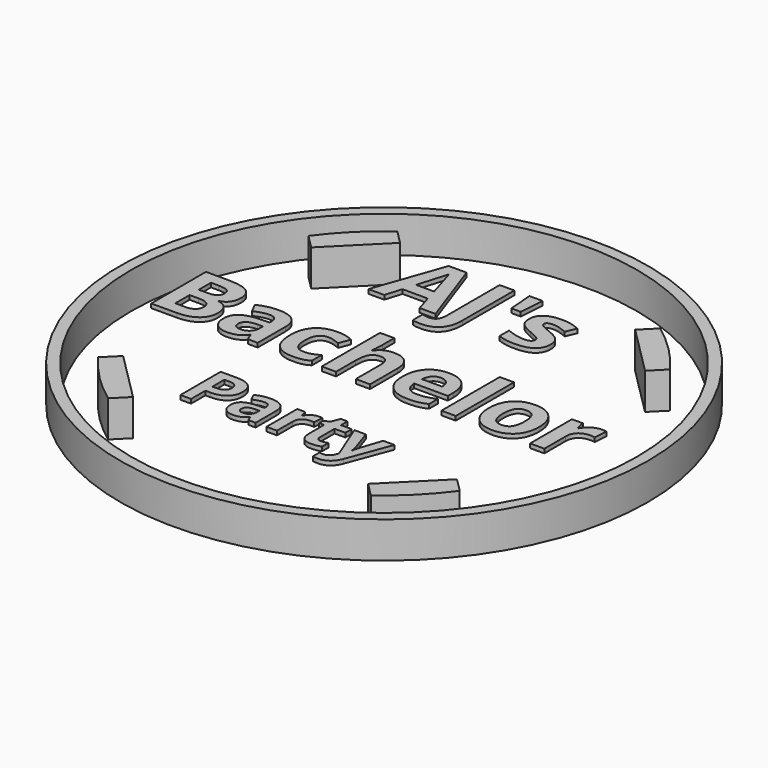
from build123d import *

# Parameters (mm, degrees)
F0_TEXT_SIZE = 8.7192851648
F1_TEXT_SIZE = 8.8355448193
F2_TEXT_SIZE = 6.411131907
F4_DEPTH     = 0.381
F5_DEPTH     = 3.302
F6_R         = 24
F6_R_2       = 23
F7_DEPTH     = 3.302


# Not quite as in the source:
# - Text() gives the source's letters only with a copy of the font that has no kerning and outlines rounded to 1/6400 em; it was checked with that copy


with BuildPart() as f4:
    # F0 (on Top) + F1 (on Top) + F2 (on Top) → F4 (new body)
    with BuildSketch(Plane.XY):
        with Locations((-19.4460495, -3.1389426593)):
            Text('Bachelor', F0_TEXT_SIZE, font='Open Sans', font_style=FontStyle.BOLD, text_align=(TextAlign.LEFT, TextAlign.BOTTOM))
    with BuildSketch(Plane.XY):
        with Locations((-8.001, 8.2189426593)):
            Text("AJ's", F1_TEXT_SIZE, font='Open Sans', font_style=FontStyle.BOLD, text_align=(TextAlign.LEFT, TextAlign.BOTTOM))
    with BuildSketch(Plane.XY):
        with Locations((-8.8278281141, -12.8349576324)):
            Text('Party', F2_TEXT_SIZE, font='Open Sans', font_style=FontStyle.BOLD, text_align=(TextAlign.LEFT, TextAlign.BOTTOM))
    extrude(amount=-F4_DEPTH)


with BuildPart() as f5:
    # F3 (on Top) → F5 (new body)
    with BuildSketch(Plane.XY):
        with BuildLine():
            Line((-16.4369943958, 11.9468663353), (-15.1766328446, 10.6865047841))
            Line((-15.1766328446, 10.6865047841), (-10.6865047841, 15.1766328446))
            Line((-10.6865047841, 15.1766328446), (-11.9468663353, 16.4369943958))
            ThreePointArc((-11.9468663353, 16.4369943958), (-14.3684097937, 14.3684097937), (-16.4369943958, 11.9468663353))
        make_face()
    extrude(amount=-F5_DEPTH)


with BuildPart() as f5b:
    # F3 (on Top) → F5, piece 2 (new body)
    with BuildSketch(Plane.XY):
        with BuildLine():
            Line((-10.6865047841, -15.1766328446), (-15.1766328446, -10.6865047841))
            Line((-15.1766328446, -10.6865047841), (-16.4369943958, -11.9468663353))
            ThreePointArc((-16.4369943958, -11.9468663353), (-14.3684097937, -14.3684097937), (-11.9468663353, -16.4369943958))
            Line((-11.9468663353, -16.4369943958), (-10.6865047841, -15.1766328446))
        make_face()
    extrude(amount=-F5_DEPTH)


with BuildPart() as f5c:
    # F3 (on Top) → F5, piece 3 (new body)
    with BuildSketch(Plane.XY):
        with BuildLine():
            Line((15.1766328446, -10.6865047841), (10.6865047841, -15.1766328446))
            Line((10.6865047841, -15.1766328446), (11.9468663353, -16.4369943958))
            ThreePointArc((11.9468663353, -16.4369943958), (14.3684097937, -14.3684097937), (16.4369943958, -11.9468663353))
            Line((16.4369943958, -11.9468663353), (15.1766328446, -10.6865047841))
        make_face()
    extrude(amount=-F5_DEPTH)


with BuildPart() as f5d:
    # F3 (on Top) → F5, piece 4 (new body)
    with BuildSketch(Plane.XY):
        with BuildLine():
            Line((10.6865047841, 15.1766328446), (15.1766328446, 10.6865047841))
            Line((15.1766328446, 10.6865047841), (16.4369943958, 11.9468663353))
            ThreePointArc((16.4369943958, 11.9468663353), (14.3684097937, 14.3684097937), (11.9468663353, 16.4369943958))
            Line((11.9468663353, 16.4369943958), (10.6865047841, 15.1766328446))
        make_face()
    extrude(amount=-F5_DEPTH)


with BuildPart() as f7:
    # F6 (on Top) → F7 (new body)
    with BuildSketch(Plane.XY):
        Circle(F6_R)
        Circle(F6_R_2, mode=Mode.SUBTRACT)
    extrude(amount=-F7_DEPTH)


solid = Compound([f4.part, f5.part, f5b.part, f5c.part, f5d.part, f7.part])
